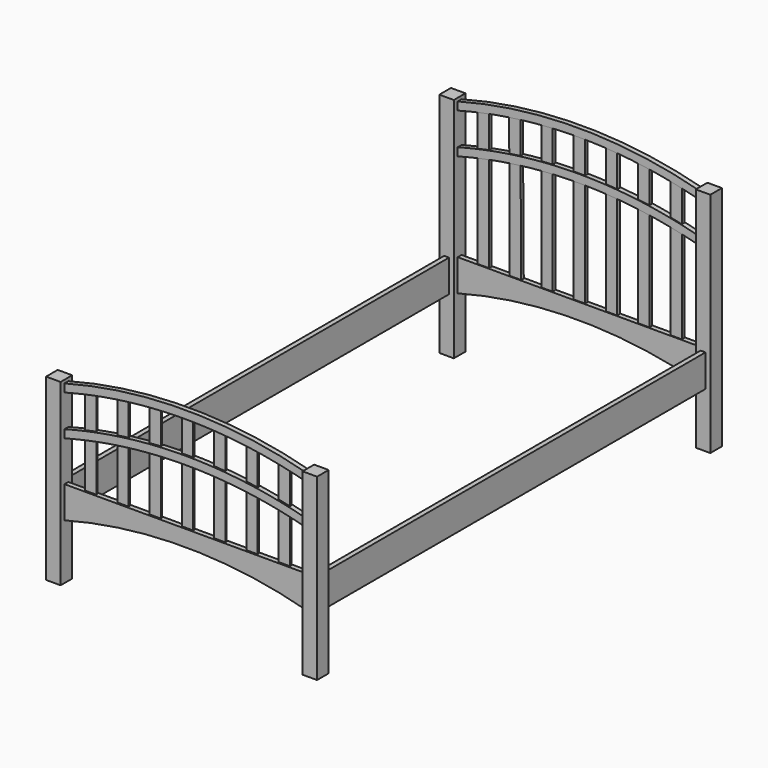
from build123d import *

# Parameters (mm, degrees)
F1_DEPTH  = 28.575
F2_DEPTH  = 9.525
F3_DEPTH  = 3.175
F6_DEPTH  = 28.575
F5_W      = 44.45
F5_H      = 15.7440634199
F5_H_2    = 14.4274564214
F5_H_3    = 10.4776354261
F5_H_4    = 13.110849423
F7_DEPTH  = 9.525
F8_DEPTH  = 6.35
F9_W      = 19.05
F9_H      = 127
F10_W     = 19.05
F10_H     = 127
F11_DEPTH = 1879.6


# Not quite as in the source:
# - a feature names something its author has since deleted; it is built from what else it names


with BuildPart() as f1:
    # F0 (on Front) → F1 (new body, symmetric)
    with BuildSketch(Plane.XZ):
        Polygon((-476.25, 352.425), (-533.4, 352.425), (-533.4, -352.425), (-476.25, -352.425), (-476.25, -134.8195257052), (-476.25, -9.525), (-476.25, 149.225), (-476.25, 180.975), (-476.25, 307.975), (-476.25, 339.725), align=None)
    extrude(amount=F1_DEPTH, both=True)



with BuildPart() as f1b:
    # F0 (on Front) → F1, piece 2 (new body, symmetric)
    with BuildSketch(Plane.XZ):
        Polygon((476.25, 352.425), (476.25, 339.725), (476.25, 307.975), (476.25, 180.975), (476.25, 149.225), (476.25, -9.525), (476.25, -136.525), (476.25, -352.425), (533.4, -352.425), (533.4, 352.425), align=None)
    extrude(amount=F1_DEPTH, both=True)


with BuildPart() as f1_1:
    add(f1.part)

    add(f1b.part)  # F2 merges F1b
    # F0 (on Front) → F2 (join, symmetric)
    with BuildSketch(Plane.XZ):
        with BuildLine():
            ThreePointArc((476.25, 339.725), (0, 402.3720732762), (-476.25, 339.725))
            Line((-476.25, 339.725), (-476.25, 307.975))
            ThreePointArc((-476.25, 307.975), (-438.2494329096, 317.7158637889), (-400.05, 326.6450771885))
            ThreePointArc((-400.05, 326.6450771885), (-377.853727219, 331.4413518638), (-355.6, 335.9635638217))
            ThreePointArc((-355.6, 335.9635638217), (-314.4063502859, 343.5848084623), (-273.05, 350.267056413))
            ThreePointArc((-273.05, 350.267056413), (-250.8436134426, 353.458212086), (-228.6, 356.3786126552))
            ThreePointArc((-228.6, 356.3786126552), (-187.3725603705, 361.0650937066), (-146.05, 364.8215398287))
            ThreePointArc((-146.05, 364.8215398287), (-123.8340593774, 366.4538372691), (-101.6, 367.8172947439))
            ThreePointArc((-101.6, 367.8172947439), (-60.3401737333, 369.6332696908), (-19.05, 370.5235402345))
            ThreePointArc((-19.05, 370.5235402345), (3.1752312419, 370.6193359197), (25.4, 370.4468997792))
            ThreePointArc((25.4, 370.4468997792), (66.6917749651, 369.4140721859), (107.95, 367.4554299056))
            ThreePointArc((107.95, 367.4554299056), (130.1845285142, 366.0148139341), (152.4, 364.3052937414))
            ThreePointArc((152.4, 364.3052937414), (193.7242080894, 360.4043394445), (234.95, 355.5730145764))
            ThreePointArc((234.95, 355.5730145764), (257.1941031877, 352.573798396), (279.4, 349.3036957855))
            ThreePointArc((279.4, 349.3036957855), (320.7580955835, 342.4727795848), (361.95, 334.7022907339))
            ThreePointArc((361.95, 334.7022907339), (384.2042536133, 330.098341116), (406.4, 325.2201244017))
            ThreePointArc((406.4, 325.2201244017), (441.4092253271, 316.9387101661), (476.25, 307.975))
            Line((476.25, 307.975), (476.25, 339.725))
        make_face()
        with BuildLine():
            ThreePointArc((-400.05, 199.6450771885), (-438.2494329096, 190.7158637889), (-476.25, 180.975))
            Line((-476.25, 180.975), (-476.25, 149.225))
            ThreePointArc((-476.25, 149.225), (-438.2494329096, 158.9658637889), (-400.05, 167.8950771885))
            ThreePointArc((-400.05, 167.8950771885), (-377.853727219, 172.6913518638), (-355.6, 177.2135638217))
            ThreePointArc((-355.6, 177.2135638217), (-314.4063502859, 184.8348084623), (-273.05, 191.517056413))
            ThreePointArc((-273.05, 191.517056413), (-250.8436134426, 194.708212086), (-228.6, 197.6286126552))
            ThreePointArc((-228.6, 197.6286126552), (-187.3725603705, 202.3150937066), (-146.05, 206.0715398287))
            ThreePointArc((-146.05, 206.0715398287), (-123.8340593774, 207.7038372691), (-101.6, 209.0672947439))
            ThreePointArc((-101.6, 209.0672947439), (-60.3401737333, 210.8832696908), (-19.05, 211.7735402345))
            ThreePointArc((-19.05, 211.7735402345), (3.1752312419, 211.8693359197), (25.4, 211.6968997792))
            ThreePointArc((25.4, 211.6968997792), (66.6917749651, 210.6640721859), (107.95, 208.7054299056))
            ThreePointArc((107.95, 208.7054299056), (130.1845285142, 207.2648139341), (152.4, 205.5552937414))
            ThreePointArc((152.4, 205.5552937414), (193.7242080894, 201.6543394445), (234.95, 196.8230145764))
            ThreePointArc((234.95, 196.8230145764), (257.1941031877, 193.823798396), (279.4, 190.5536957855))
            ThreePointArc((279.4, 190.5536957855), (320.7580955835, 183.7227795848), (361.95, 175.9522907339))
            ThreePointArc((361.95, 175.9522907339), (384.2042536133, 171.348341116), (406.4, 166.4701244017))
            ThreePointArc((406.4, 166.4701244017), (441.4092253271, 158.1887101662), (476.25, 149.225))
            Line((476.25, 149.225), (476.25, 180.975))
            ThreePointArc((476.25, 180.975), (441.4092253271, 189.9387101661), (406.4, 198.2201244017))
            ThreePointArc((406.4, 198.2201244017), (384.2042536133, 203.098341116), (361.95, 207.7022907339))
            ThreePointArc((361.95, 207.7022907339), (320.7580955835, 215.4727795848), (279.4, 222.3036957855))
            ThreePointArc((279.4, 222.3036957855), (257.1941031877, 225.573798396), (234.95, 228.5730145764))
            ThreePointArc((234.95, 228.5730145764), (193.7242080894, 233.4043394445), (152.4, 237.3052937414))
            ThreePointArc((152.4, 237.3052937414), (130.1845285142, 239.0148139341), (107.95, 240.4554299056))
            ThreePointArc((107.95, 240.4554299056), (66.6917749651, 242.4140721859), (25.4, 243.4468997792))
            ThreePointArc((25.4, 243.4468997792), (3.1752312419, 243.6193359197), (-19.05, 243.5235402345))
            ThreePointArc((-19.05, 243.5235402345), (-60.3401737333, 242.6332696908), (-101.6, 240.8172947439))
            ThreePointArc((-101.6, 240.8172947439), (-123.8340593774, 239.4538372691), (-146.05, 237.8215398287))
            ThreePointArc((-146.05, 237.8215398287), (-187.3725603705, 234.0650937066), (-228.6, 229.3786126552))
            ThreePointArc((-228.6, 229.3786126552), (-250.8436134426, 226.458212086), (-273.05, 223.267056413))
            ThreePointArc((-273.05, 223.267056413), (-314.4063502859, 216.5848084623), (-355.6, 208.9635638217))
            ThreePointArc((-355.6, 208.9635638217), (-377.853727219, 204.4413518638), (-400.05, 199.6450771885))
        make_face()
        with BuildLine():
            Line((-476.25, -9.525), (-476.25, -134.8195257052))
            ThreePointArc((-476.25, -134.8195257052), (0.1121710863, -73.0251974288), (476.25, -136.525))
            Line((476.25, -136.525), (476.25, -9.525))
            Line((476.25, -9.525), (406.4, -9.525))
            Line((406.4, -9.525), (361.95, -9.525))
            Line((361.95, -9.525), (279.4, -9.525))
            Line((279.4, -9.525), (234.95, -9.525))
            Line((234.95, -9.525), (152.4, -9.525))
            Line((152.4, -9.525), (107.95, -9.525))
            Line((107.95, -9.525), (25.4, -9.525))
            Line((25.4, -9.525), (-19.05, -9.525))
            Line((-19.05, -9.525), (-101.6, -9.525))
            Line((-101.6, -9.525), (-146.05, -9.525))
            Line((-146.05, -9.525), (-228.6, -9.525))
            Line((-228.6, -9.525), (-273.05, -9.525))
            Line((-273.05, -9.525), (-355.6, -9.525))
            Line((-355.6, -9.525), (-400.05, -9.525))
            Line((-400.05, -9.525), (-476.25, -9.525))
        make_face()
    extrude(amount=F2_DEPTH, both=True)

    # F0 (on Front) → F3 (join, symmetric)
    with BuildSketch(Plane.XZ):
        with BuildLine():
            Line((-400.05, 167.8950771885), (-400.05, -9.525))
            Line((-400.05, -9.525), (-355.6, -9.525))
            Line((-355.6, -9.525), (-355.6, 177.2135638217))
            ThreePointArc((-355.6, 177.2135638217), (-377.853727219, 172.6913518638), (-400.05, 167.8950771885))
        make_face()
        with BuildLine():
            Line((-273.05, 191.517056413), (-273.05, -9.525))
            Line((-273.05, -9.525), (-228.6, -9.525))
            Line((-228.6, -9.525), (-228.6, 197.6286126552))
            ThreePointArc((-228.6, 197.6286126552), (-250.8436134426, 194.708212086), (-273.05, 191.517056413))
        make_face()
        with BuildLine():
            ThreePointArc((-355.6, 335.9635638217), (-377.853727219, 331.4413518638), (-400.05, 326.6450771885))
            Line((-400.05, 326.6450771885), (-400.05, 199.6450771885))
            ThreePointArc((-400.05, 199.6450771885), (-377.853727219, 204.4413518638), (-355.6, 208.9635638217))
            Line((-355.6, 208.9635638217), (-355.6, 335.9635638217))
        make_face()
        with BuildLine():
            ThreePointArc((-228.6, 356.3786126552), (-250.8436134426, 353.458212086), (-273.05, 350.267056413))
            Line((-273.05, 350.267056413), (-273.05, 223.267056413))
            ThreePointArc((-273.05, 223.267056413), (-250.8436134426, 226.458212086), (-228.6, 229.3786126552))
            Line((-228.6, 229.3786126552), (-228.6, 356.3786126552))
        make_face()
        with BuildLine():
            ThreePointArc((-101.6, 367.8172947439), (-123.8340593774, 366.4538372691), (-146.05, 364.8215398287))
            Line((-146.05, 364.8215398287), (-146.05, 237.8215398287))
            ThreePointArc((-146.05, 237.8215398287), (-123.8340593774, 239.4538372691), (-101.6, 240.8172947439))
            Line((-101.6, 240.8172947439), (-101.6, 367.8172947439))
        make_face()
        with BuildLine():
            Line((-146.05, 206.0715398287), (-146.05, -9.525))
            Line((-146.05, -9.525), (-101.6, -9.525))
            Line((-101.6, -9.525), (-101.6, 209.0672947439))
            ThreePointArc((-101.6, 209.0672947439), (-123.8340593774, 207.7038372691), (-146.05, 206.0715398287))
        make_face()
        with BuildLine():
            Line((-19.05, 211.7735402345), (-19.05, -9.525))
            Line((-19.05, -9.525), (25.4, -9.525))
            Line((25.4, -9.525), (25.4, 211.6968997792))
            ThreePointArc((25.4, 211.6968997792), (3.1752312419, 211.8693359197), (-19.05, 211.7735402345))
        make_face()
        with BuildLine():
            ThreePointArc((25.4, 370.4468997792), (3.1752312419, 370.6193359197), (-19.05, 370.5235402345))
            Line((-19.05, 370.5235402345), (-19.05, 243.5235402345))
            ThreePointArc((-19.05, 243.5235402345), (3.1752312419, 243.6193359197), (25.4, 243.4468997792))
            Line((25.4, 243.4468997792), (25.4, 370.4468997792))
        make_face()
        with BuildLine():
            Line((152.4, 237.3052937414), (152.4, 364.3052937414))
            ThreePointArc((152.4, 364.3052937414), (130.1845285142, 366.0148139341), (107.95, 367.4554299056))
            Line((107.95, 367.4554299056), (107.95, 240.4554299056))
            ThreePointArc((107.95, 240.4554299056), (130.1845285142, 239.0148139341), (152.4, 237.3052937414))
        make_face()
        with BuildLine():
            Line((107.95, -9.525), (152.4, -9.525))
            Line((152.4, -9.525), (152.4, 205.5552937414))
            ThreePointArc((152.4, 205.5552937414), (130.1845285142, 207.2648139341), (107.95, 208.7054299056))
            Line((107.95, 208.7054299056), (107.95, -9.525))
        make_face()
        with BuildLine():
            Line((234.95, -9.525), (279.4, -9.525))
            Line((279.4, -9.525), (279.4, 190.5536957855))
            ThreePointArc((279.4, 190.5536957855), (257.1941031877, 193.823798396), (234.95, 196.8230145764))
            Line((234.95, 196.8230145764), (234.95, -9.525))
        make_face()
        with BuildLine():
            Line((279.4, 222.3036957855), (279.4, 349.3036957855))
            ThreePointArc((279.4, 349.3036957855), (257.1941031877, 352.573798396), (234.95, 355.5730145764))
            Line((234.95, 355.5730145764), (234.95, 228.5730145764))
            ThreePointArc((234.95, 228.5730145764), (257.1941031877, 225.573798396), (279.4, 222.3036957855))
        make_face()
        with BuildLine():
            Line((406.4, 198.2201244017), (406.4, 325.2201244017))
            ThreePointArc((406.4, 325.2201244017), (384.2042536133, 330.098341116), (361.95, 334.7022907339))
            Line((361.95, 334.7022907339), (361.95, 207.7022907339))
            ThreePointArc((361.95, 207.7022907339), (384.2042536133, 203.098341116), (406.4, 198.2201244017))
        make_face()
        with BuildLine():
            Line((361.95, -9.525), (406.4, -9.525))
            Line((406.4, -9.525), (406.4, 166.4701244017))
            ThreePointArc((406.4, 166.4701244017), (384.2042536133, 171.348341116), (361.95, 175.9522907339))
            Line((361.95, 175.9522907339), (361.95, -9.525))
        make_face()
    extrude(amount=F3_DEPTH, both=True)



with BuildPart() as f6:
    # F5 (on offset) → F6 (new body, symmetric)
    with BuildSketch(Plane.XZ.offset(-1935.1498)):
        Polygon((-476.25, 542.925), (-533.4, 542.925), (-533.4, -352.425), (-476.25, -352.425), (-476.25, -134.8195257053), (-476.25, -9.525), (-476.25, 339.725), (-476.25, 371.475), (-476.25, 498.475), (-476.25, 530.225), align=None)
    extrude(amount=F6_DEPTH, both=True)



with BuildPart() as f6b:
    # F5 (on offset) → F6, piece 2 (new body, symmetric)
    with BuildSketch(Plane.XZ.offset(-1935.1498)):
        Polygon((476.25, 542.925), (476.25, 530.225), (476.25, 498.475), (476.25, 371.475), (476.25, 339.725), (476.25, -9.525), (476.25, -136.525), (476.25, -352.425), (533.4, -352.425), (533.4, 542.925), align=None)
    extrude(amount=F6_DEPTH, both=True)


with BuildPart() as f6_1:
    add(f6.part)

    add(f6b.part)  # F7 merges F6b
    # F5 (on offset) → F7 (join, symmetric)
    with BuildSketch(Plane.XZ.offset(-1935.1498)):
        with BuildLine():
            ThreePointArc((-400.05, 390.1450771885), (-438.2494329096, 381.2158637889), (-476.25, 371.475))
            Line((-476.25, 371.475), (-476.25, 339.725))
            ThreePointArc((-476.25, 339.725), (-438.2494329096, 349.4658637889), (-400.05, 358.3950771885))
            ThreePointArc((-400.05, 358.3950771885), (-377.853727219, 363.1913518638), (-355.6, 367.7135638217))
            ThreePointArc((-355.6, 367.7135638217), (-315.7526382333, 375.1010217711), (-275.7523639485, 381.6098489978))
            ThreePointArc((-275.7523639485, 381.6098489978), (-253.5731226042, 384.830843308), (-231.356325078, 387.7816836351))
            ThreePointArc((-231.356325078, 387.7816836351), (-190.3385028325, 392.5093210474), (-149.225, 396.3161809223))
            ThreePointArc((-149.225, 396.3161809223), (-127.009293862, 397.987082617), (-104.775, 399.3891126256))
            ThreePointArc((-104.775, 399.3891126256), (-63.5159742062, 401.2764141749), (-22.225, 402.2379575627))
            ThreePointArc((-22.225, 402.2379575627), (0, 402.3720732762), (22.225, 402.2379575627))
            ThreePointArc((22.225, 402.2379575627), (63.5159742062, 401.2764141749), (104.775, 399.3891126256))
            ThreePointArc((104.775, 399.3891126256), (127.009293862, 397.987082617), (149.225, 396.3161809223))
            ThreePointArc((149.225, 396.3161809223), (190.5483837871, 392.4874995721), (231.775, 387.7286169155))
            ThreePointArc((231.775, 387.7286169155), (254.0188581392, 384.7688226688), (276.225, 381.5382080895))
            ThreePointArc((276.225, 381.5382080895), (317.5822221474, 374.781659489), (358.775, 367.0858277911))
            ThreePointArc((358.775, 367.0858277911), (381.0289901299, 362.5227696417), (403.225, 357.6855470685))
            ThreePointArc((403.225, 357.6855470685), (439.8291875478, 349.0780619107), (476.25, 339.725))
            Line((476.25, 339.725), (476.25, 371.475))
            ThreePointArc((476.25, 371.475), (439.8291875478, 380.8280619107), (403.225, 389.4355470685))
            ThreePointArc((403.225, 389.4355470685), (381.0289901299, 394.2727696417), (358.775, 398.8358277911))
            ThreePointArc((358.775, 398.8358277911), (317.5822221474, 406.531659489), (276.225, 413.2882080895))
            ThreePointArc((276.225, 413.2882080895), (254.0188581392, 416.5188226688), (231.775, 419.4786169155))
            ThreePointArc((231.775, 419.4786169155), (190.5483837871, 424.2374995721), (149.225, 428.0661809223))
            ThreePointArc((149.225, 428.0661809223), (127.009293862, 429.737082617), (104.775, 431.1391126256))
            ThreePointArc((104.775, 431.1391126256), (63.5159742062, 433.0264141749), (22.225, 433.9879575627))
            ThreePointArc((22.225, 433.9879575627), (0, 434.1220732762), (-22.225, 433.9879575627))
            ThreePointArc((-22.225, 433.9879575627), (-63.5159742062, 433.0264141749), (-104.775, 431.1391126256))
            ThreePointArc((-104.775, 431.1391126256), (-127.009293862, 429.737082617), (-149.225, 428.0661809223))
            ThreePointArc((-149.225, 428.0661809223), (-190.4374228458, 424.2490392903), (-231.5536536851, 419.5066845339))
            ThreePointArc((-231.5536536851, 419.5066845339), (-253.7189748289, 416.5605613251), (-275.8468911887, 413.3455308519))
            ThreePointArc((-275.8468911887, 413.3455308519), (-315.7997329798, 406.842825006), (-355.6, 399.4635638217))
            ThreePointArc((-355.6, 399.4635638217), (-377.853727219, 394.9413518638), (-400.05, 390.1450771885))
        make_face()
        with BuildLine():
            ThreePointArc((476.25, 530.225), (0, 592.8720732762), (-476.25, 530.225))
            Line((-476.25, 530.225), (-476.25, 498.475))
            ThreePointArc((-476.25, 498.475), (-438.2494329096, 508.2158637889), (-400.05, 517.1450771885))
            ThreePointArc((-400.05, 517.1450771885), (-377.853727219, 521.9413518638), (-355.6, 526.4635638217))
            ThreePointArc((-355.6, 526.4635638217), (-315.9881134687, 533.8100250889), (-276.225, 540.2882080895))
            ThreePointArc((-276.225, 540.2882080895), (-254.3023839705, 543.4793144722), (-232.3429667677, 546.4064717346))
            ThreePointArc((-232.3429667677, 546.4064717346), (-190.833110221, 551.2078574997), (-149.225, 555.0661809223))
            ThreePointArc((-149.225, 555.0661809223), (-127.009293862, 556.737082617), (-104.775, 558.1391126256))
            ThreePointArc((-104.775, 558.1391126256), (-63.5159742062, 560.0264141749), (-22.225, 560.9879575627))
            ThreePointArc((-22.225, 560.9879575627), (0, 561.1220732762), (22.225, 560.9879575627))
            ThreePointArc((22.225, 560.9879575627), (63.5159742062, 560.0264141749), (104.775, 558.1391126256))
            ThreePointArc((104.775, 558.1391126256), (127.009293862, 556.737082617), (149.225, 555.0661809223))
            ThreePointArc((149.225, 555.0661809223), (190.5483837871, 551.2374995721), (231.775, 546.4786169155))
            ThreePointArc((231.775, 546.4786169155), (254.0188581392, 543.5188226688), (276.225, 540.2882080895))
            ThreePointArc((276.225, 540.2882080895), (317.5822221474, 533.531659489), (358.775, 525.8358277911))
            ThreePointArc((358.775, 525.8358277911), (381.0289901299, 521.2727696417), (403.225, 516.4355470685))
            ThreePointArc((403.225, 516.4355470685), (439.8291875478, 507.8280619107), (476.25, 498.475))
            Line((476.25, 498.475), (476.25, 530.225))
        make_face()
        Polygon((-228.8850887576, -9.525), (-274.5873378436, -9.525), (-274.4508164136, -55.3594140888), (-228.6, -55.3594140888), align=None)
        Polygon((-355.6, -9.525), (-400.05, -9.525), (-355.6, -55.3594140888), align=None)
        with Locations((-127, -17.3970317099)):
            Rectangle(F5_W, F5_H)
        with Locations((0, -16.7387282107)):
            Rectangle(F5_W, F5_H_2)
        with Locations((127, -14.7638177131)):
            Rectangle(F5_W, F5_H_3)
        with Locations((254, -16.0804247115)):
            Rectangle(F5_W, F5_H_4)
        with Locations((381, -17.3970317099)):
            Rectangle(F5_W, F5_H)
        with BuildLine():
            Line((-476.25, -9.525), (-476.25, -134.8195257053))
            ThreePointArc((-476.25, -134.8195257052), (0.1121710863, -73.0251974288), (476.25, -136.525))
            Line((476.25, -136.525), (476.25, -9.525))
            Line((476.25, -9.525), (403.225, -9.525))
            Line((403.225, -9.525), (403.225, -25.2690634199))
            Line((403.225, -25.2690634199), (358.775, -25.2690634199))
            Line((358.775, -25.2690634199), (358.775, -9.525))
            Line((358.775, -9.525), (276.225, -9.525))
            Line((276.225, -9.525), (276.225, -22.635849423))
            Line((276.225, -22.635849423), (231.775, -22.635849423))
            Line((231.775, -22.635849423), (231.775, -9.525))
            Line((231.775, -9.525), (149.225, -9.525))
            Line((149.225, -9.525), (149.225, -20.0026354261))
            Line((149.225, -20.0026354261), (104.775, -20.0026354261))
            Line((104.775, -20.0026354261), (104.775, -9.525))
            Line((104.775, -9.525), (22.225, -9.525))
            Line((22.225, -9.525), (22.225, -23.9524564214))
            Line((22.225, -23.9524564214), (-22.225, -23.9524564214))
            Line((-22.225, -23.9524564214), (-22.225, -9.525))
            Line((-22.225, -9.525), (-104.775, -9.525))
            Line((-104.775, -9.525), (-104.775, -25.2690634199))
            Line((-104.775, -25.2690634199), (-149.225, -25.2690634199))
            Line((-149.225, -25.2690634199), (-149.225, -9.525))
            Line((-149.225, -9.525), (-228.8850887576, -9.525))
            Line((-228.8850887576, -9.525), (-228.6, -55.3594140888))
            Line((-228.6, -55.3594140888), (-274.4508164136, -55.3594140888))
            Line((-274.4508164136, -55.3594140888), (-274.5873378436, -9.525))
            Line((-274.5873378436, -9.525), (-355.6, -9.525))
            Line((-355.6, -9.525), (-355.6, -55.3594140888))
            Line((-355.6, -55.3594140888), (-400.05, -9.525))
            Line((-400.05, -9.525), (-476.25, -9.525))
        make_face()
    extrude(amount=F7_DEPTH, both=True)

    # F5 (on offset) → F8 (join, symmetric)
    with BuildSketch(Plane.XZ.offset(-1935.1498)):
        with BuildLine():
            Line((-400.05, 358.3950771885), (-400.05, -9.525))
            Line((-400.05, -9.525), (-355.6, -9.525))
            Line((-355.6, -9.525), (-355.6, 367.7135638217))
            ThreePointArc((-355.6, 367.7135638217), (-377.853727219, 363.1913518638), (-400.05, 358.3950771885))
        make_face()
        with BuildLine():
            ThreePointArc((-355.6, 526.4635638217), (-377.853727219, 521.9413518638), (-400.05, 517.1450771885))
            Line((-400.05, 517.1450771885), (-400.05, 390.1450771885))
            ThreePointArc((-400.05, 390.1450771885), (-377.853727219, 394.9413518638), (-355.6, 399.4635638217))
            Line((-355.6, 399.4635638217), (-355.6, 526.4635638217))
        make_face()
        with BuildLine():
            ThreePointArc((-232.3429667677, 546.4064717346), (-254.3023839705, 543.4793144722), (-276.225, 540.2882080895))
            Line((-276.225, 540.2882080895), (-275.8468911887, 413.3455308519))
            ThreePointArc((-275.8468911887, 413.3455308519), (-253.7189748289, 416.5605613251), (-231.5536536851, 419.5066845339))
            Line((-231.5536536851, 419.5066845339), (-232.3429667677, 546.4064717346))
        make_face()
        with BuildLine():
            Line((-275.7523639485, 381.6098489978), (-274.5873378436, -9.525))
            Line((-274.5873378436, -9.525), (-228.8850887576, -9.525))
            Line((-228.8850887576, -9.525), (-231.356325078, 387.7816836351))
            ThreePointArc((-231.356325078, 387.7816836351), (-253.5731226042, 384.830843308), (-275.7523639485, 381.6098489978))
        make_face()
        with BuildLine():
            Line((-149.225, 396.3161809223), (-149.225, -9.525))
            Line((-149.225, -9.525), (-104.775, -9.525))
            Line((-104.775, -9.525), (-104.775, 399.3891126256))
            ThreePointArc((-104.775, 399.3891126256), (-127.009293862, 397.987082617), (-149.225, 396.3161809223))
        make_face()
        with BuildLine():
            ThreePointArc((-104.775, 558.1391126256), (-127.009293862, 556.737082617), (-149.225, 555.0661809223))
            Line((-149.225, 555.0661809223), (-149.225, 428.0661809223))
            ThreePointArc((-149.225, 428.0661809223), (-127.009293862, 429.737082617), (-104.775, 431.1391126256))
            Line((-104.775, 431.1391126256), (-104.775, 558.1391126256))
        make_face()
        with BuildLine():
            ThreePointArc((22.225, 560.9879575627), (0, 561.1220732762), (-22.225, 560.9879575627))
            Line((-22.225, 560.9879575627), (-22.225, 433.9879575627))
            ThreePointArc((-22.225, 433.9879575627), (0, 434.1220732762), (22.225, 433.9879575627))
            Line((22.225, 433.9879575627), (22.225, 560.9879575627))
        make_face()
        with BuildLine():
            Line((-22.225, 402.2379575627), (-22.225, -9.525))
            Line((-22.225, -9.525), (22.225, -9.525))
            Line((22.225, -9.525), (22.225, 402.2379575627))
            ThreePointArc((22.225, 402.2379575627), (0, 402.3720732762), (-22.225, 402.2379575627))
        make_face()
        with BuildLine():
            Line((104.775, -9.525), (149.225, -9.525))
            Line((149.225, -9.525), (149.225, 396.3161809223))
            ThreePointArc((149.225, 396.3161809223), (127.009293862, 397.987082617), (104.775, 399.3891126256))
            Line((104.775, 399.3891126256), (104.775, -9.525))
        make_face()
        with BuildLine():
            Line((149.225, 428.0661809223), (149.225, 555.0661809223))
            ThreePointArc((149.225, 555.0661809223), (127.009293862, 556.737082617), (104.775, 558.1391126256))
            Line((104.775, 558.1391126256), (104.775, 431.1391126256))
            ThreePointArc((104.775, 431.1391126256), (127.009293862, 429.737082617), (149.225, 428.0661809223))
        make_face()
        with BuildLine():
            Line((231.775, -9.525), (276.225, -9.525))
            Line((276.225, -9.525), (276.225, 381.5382080895))
            ThreePointArc((276.225, 381.5382080895), (254.0188581392, 384.7688226688), (231.775, 387.7286169155))
            Line((231.775, 387.7286169155), (231.775, -9.525))
        make_face()
        with BuildLine():
            Line((276.225, 413.2882080895), (276.225, 540.2882080895))
            ThreePointArc((276.225, 540.2882080895), (254.0188581392, 543.5188226688), (231.775, 546.4786169155))
            Line((231.775, 546.4786169155), (231.775, 419.4786169155))
            ThreePointArc((231.775, 419.4786169155), (254.0188581392, 416.5188226688), (276.225, 413.2882080895))
        make_face()
        with BuildLine():
            Line((403.225, 389.4355470685), (403.225, 516.4355470685))
            ThreePointArc((403.225, 516.4355470685), (381.0289901299, 521.2727696417), (358.775, 525.8358277911))
            Line((358.775, 525.8358277911), (358.775, 398.8358277911))
            ThreePointArc((358.775, 398.8358277911), (381.0289901299, 394.2727696417), (403.225, 389.4355470685))
        make_face()
        with BuildLine():
            Line((358.775, -9.525), (403.225, -9.525))
            Line((403.225, -9.525), (403.225, 357.6855470685))
            ThreePointArc((403.225, 357.6855470685), (381.0289901299, 362.5227696417), (358.775, 367.0858277911))
            Line((358.775, 367.0858277911), (358.775, -9.525))
        make_face()
    extrude(amount=F8_DEPTH, both=True)


with BuildPart() as f1_2:
    add(f1_1.part)

    add(f6_1.part)  # F11 merges F6
    # F9 (on face) + F10 (on face) → F11 (join)
    with BuildSketch(Plane.XZ.offset(-1906.5748)):
        with Locations((504.825, -73.025)):
            Rectangle(F9_W, F9_H)
    with BuildSketch(Plane.XZ.offset(-1906.5748)):
        with Locations((-504.825, -73.025)):
            Rectangle(F10_W, F10_H)
    extrude(amount=F11_DEPTH)


solid = f1_2.part
